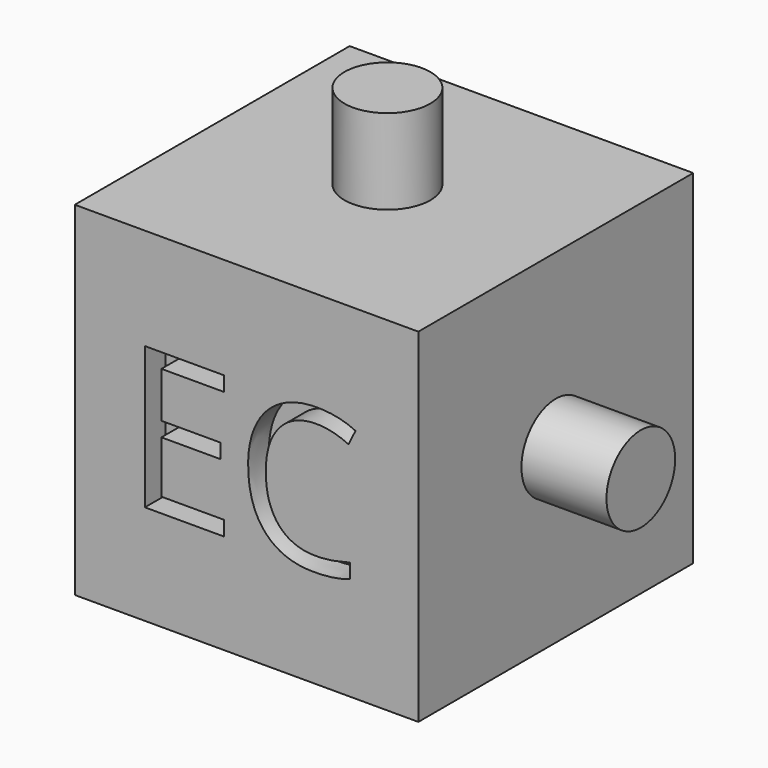
from build123d import *

# Parameters (mm, degrees)
F0_W         = 40
F0_H         = 40
F1_DEPTH     = 40
F2_TEXT_SIZE = 23.1523726446
F3_DEPTH     = 3
F4_R         = 5
F5_DEPTH     = 9.9
F6_R         = 5
F7_DEPTH     = 9.9
F8_R         = 5
F9_DEPTH     = 9.9
F10_R        = 5
F11_DEPTH    = 9.9


# Not quite as in the source:
# - Text() gives the source's letters only with a copy of the font that has no kerning and outlines rounded to 1/6400 em; it was checked with that copy


with BuildPart() as f1:
    # F0 (on Front) → F1 (new body)
    with BuildSketch(Plane.XZ):
        with Locations((20, 20)):
            Rectangle(F0_W, F0_H)
    extrude(amount=F1_DEPTH)

    # F2 (on face) → F3 (cut)
    with BuildSketch(Plane.XZ.offset(40)):
        with Locations((5.8918802533, 11.6400541738)):
            Text('EC', F2_TEXT_SIZE, font='Open Sans', text_align=(TextAlign.LEFT, TextAlign.BOTTOM))
    extrude(amount=-F3_DEPTH, mode=Mode.SUBTRACT)

    # F4 (on face) → F5 (join)
    with BuildSketch(Plane(origin=(0, 0, 0), x_dir=(0, -1, 0), z_dir=(-1, 0, 0))):
        with Locations((20, 20)):
            Circle(F4_R)
    extrude(amount=F5_DEPTH)

    # F6 (on face) → F7 (join)
    with BuildSketch(Plane.YZ.offset(40)):
        with Locations((-20, 20)):
            Circle(F6_R)
    extrude(amount=F7_DEPTH)

    # F8 (on face) → F9 (join)
    with BuildSketch(Plane.XY.offset(40)):
        with Locations((19.6875017136, -19.1126838326)):
            Circle(F8_R)
    extrude(amount=F9_DEPTH)

    # F10 (on face) → F11 (join)
    with BuildSketch(Plane(origin=(0, 0, 0), x_dir=(1, 0, 0), z_dir=(0, 0, -1))):
        with Locations((20, 20)):
            Circle(F10_R)
    extrude(amount=F11_DEPTH)


solid = f1.part
